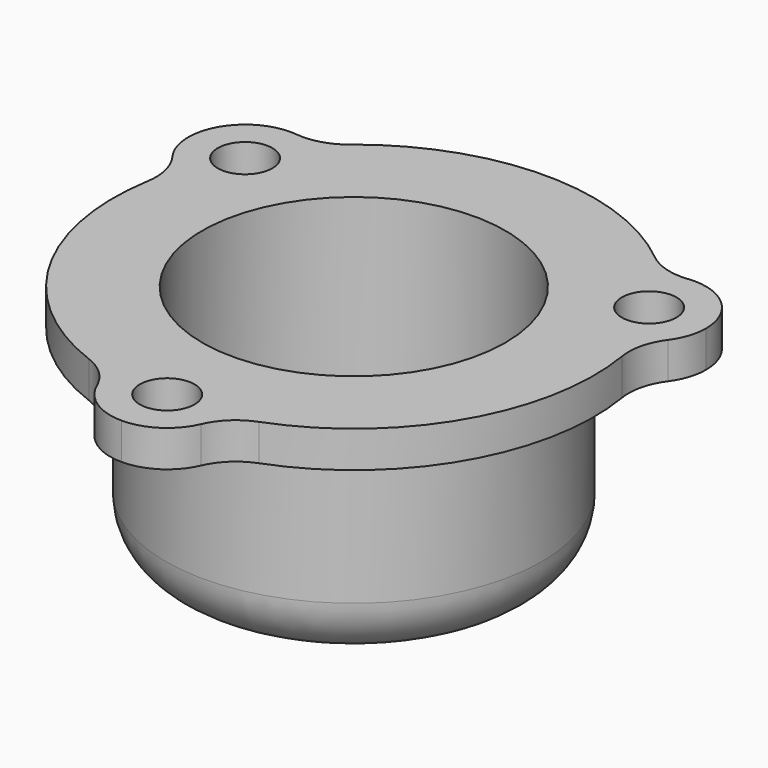
from build123d import *

# Parameters (mm, degrees)
F1_W     = 8.89
F1_H     = 3.175
F3_R     = 2.38125
F4_DEPTH = 3.176
F7_DEPTH = 3.176
F8_R     = 5.08


# Not quite as in the source:
# - a fillet or chamfer that OpenCascade refuses, or shapes differently, is made with other operations: its cross-section is extruded or revolved along the edge and cut away or added


with BuildPart() as f2:
    # F1 (on Front) → F2 (revolve)
    with BuildSketch(Plane.XZ):
        with BuildLine():
            ThreePointArc((13.208, -11.9177163316), (13.0652297207, -14.7887805254), (12.3057501177, -17.5612494052))
            Line((12.3057501177, -17.5612494052), (16.383, -17.5612494052))
            Line((16.383, -17.5612494052), (16.383, 0))
            Line((16.383, 0), (16.383, 3.175))
            Line((16.383, 3.175), (13.208, 3.175))
            Line((13.208, 3.175), (13.208, -11.9177163316))
        make_face()
        with Locations((20.828, 1.5875)):
            Rectangle(F1_W, F1_H)
    revolve(axis=Axis((0, 0, -9.4681101426), (0, 0, 1)))

    # F3 (on face) → F4 (cut, through all)
    with BuildSketch(Plane(origin=(0, 0, 0), x_dir=(1, 0, 0), z_dir=(0, 0, -1))):
        with BuildLine():
            ThreePointArc((0, 17.93875), (1.6837980227, 18.6362019773), (2.38125, 20.32))
            ThreePointArc((2.38125, 20.32), (-1.6837980227, 22.0037980227), (0, 17.93875))
        make_face()
        with Locations((-17.5976362049, -10.16)):
            Circle(F3_R)
        with Locations((17.5976362049, -10.16)):
            Circle(F3_R)
    extrude(amount=-F4_DEPTH, mode=Mode.SUBTRACT)

    # F5: fillet of radius 5.08 on 1 edges, made by hand

    # F5_s1 → F5_t2 (revolve, cut)
    with BuildSketch(Plane.XZ):
        with BuildLine():
            ThreePointArc((12.3057501177, -17.5612494052), (15.2336723724, -15.7993073042), (16.383, -12.5811999876))
            Line((16.383, -12.5811999876), (16.383, -17.5612494052))
            Line((16.383, -17.5612494052), (12.3057501177, -17.5612494052))
        make_face()
    revolve(axis=Axis((0, 0, -17.5612494052), (0, 0, 1)), mode=Mode.SUBTRACT)

    # F6 (on face) → F7 (cut, through all)
    with BuildSketch(Plane(origin=(0, 0, 0), x_dir=(1, 0, 0), z_dir=(0, 0, -1))):
        with BuildLine():
            ThreePointArc((-4.952964542, 20.3387415379), (-3.495667473, 23.8289197652), (0, 25.273))
            ThreePointArc((0, 25.273), (-21.8870601005, 12.6364998776), (-21.8870598885, -12.6365002448))
            ThreePointArc((-21.8870598885, -12.6365002448), (-22.3842836342, -8.8871231844), (-20.0903491238, -5.8799776515))
            ThreePointArc((-20.0903491238, -5.8799776515), (-18.1286292594, 10.4665689829), (-4.952964542, 20.3387415379))
        make_face()
        with BuildLine():
            ThreePointArc((0, 25.273), (3.495667473, 23.8289197652), (4.952964542, 20.3387415379))
            ThreePointArc((4.952964542, 20.3387415379), (18.1286292594, 10.4665689829), (20.0903491238, -5.8799776515))
            ThreePointArc((20.0903491238, -5.8799776515), (21.8917377458, -7.6916197707), (22.5506362049, -10.16))
            ThreePointArc((22.5506362049, -10.16), (22.3818668231, -11.4419307281), (21.8870600322, -12.6364999959))
            ThreePointArc((21.8870600322, -12.6364999959), (24.4118434084, -6.5411337246), (25.273, 0))
            ThreePointArc((25.273, 0), (17.8707096809, 17.8707096809), (0, 25.273))
        make_face()
        with BuildLine():
            ThreePointArc((-15.1373845818, -14.4587638864), (-18.8886159884, -14.9417967542), (-21.8870598885, -12.6365002448))
            ThreePointArc((-21.8870598885, -12.6365002448), (1.437e-07, -25.273), (21.8870600322, -12.6364999959))
            ThreePointArc((21.8870600322, -12.6364999959), (18.8886161272, -14.9417967167), (15.1373845818, -14.4587638864))
            ThreePointArc((15.1373845818, -14.4587638864), (0, -20.9331379659), (-15.1373845818, -14.4587638864))
        make_face()
    extrude(amount=-F7_DEPTH, mode=Mode.SUBTRACT)

    # F8
    f8_edges = [f2.edges().sort_by_distance(p)[0] for p in [
        (-15.137385, 14.458764, 1.5875),
        (15.137385, 14.458764, 1.5875),
        (20.090349, 5.879978, 1.5875),
        (4.952965, -20.338742, 1.5875),
        (-4.952965, -20.338742, 1.5875),
        (-20.090349, 5.879978, 1.5875),
    ]]
    fillet(f8_edges, radius=F8_R)


solid = f2.part
